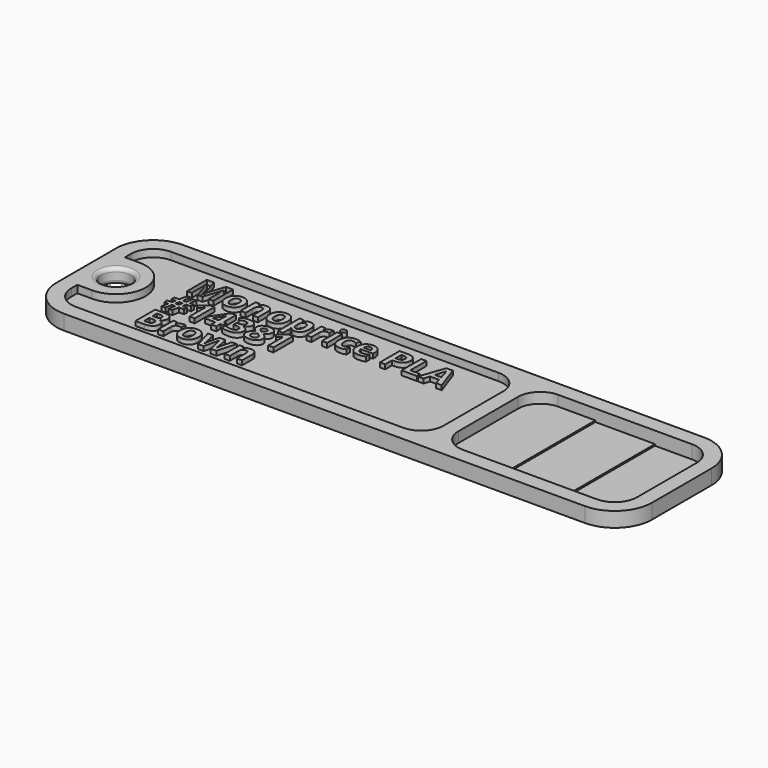
from build123d import *

# Parameters (mm, degrees)
F1_DEPTH      = 2
F3_DEPTH      = 1
F4_R          = 2
F5_DEPTH      = 2.001
F6_R          = 0.5
F7_DEPTH      = 0.4
F9_DEPTH      = 0.2
F11_DEPTH     = 0.2
F12_TEXT_SIZE = 4.6296296296
F13_DEPTH     = 0.6


# Not quite as in the source:
# - Text() gives the source's letters only with a copy of the font that has no kerning and outlines rounded to 1/6400 em; it was checked with that copy


with BuildPart() as f1:
    # F0 (on Top) → F1 (new body)
    with BuildSketch(Plane.XY):
        with BuildLine():
            ThreePointArc((40, 5), (38.5355339059, 8.5355339059), (35, 10))
            Line((35, 10), (-35, 10))
            ThreePointArc((-35, 10), (-38.5355339059, 8.5355339059), (-40, 5))
            Line((-40, 5), (-40, -5))
            ThreePointArc((-40, -5), (-38.5355339059, -8.5355339059), (-35, -10))
            Line((-35, -10), (35, -10))
            ThreePointArc((35, -10), (38.5355339059, -8.5355339059), (40, -5))
            Line((40, -5), (40, 5))
        make_face()
    extrude(amount=F1_DEPTH)

    # F2 (on face) → F3 (cut)
    with BuildSketch(Plane.XY.offset(2)):
        with BuildLine():
            ThreePointArc((35, -8), (37.1213203436, -7.1213203436), (38, -5))
            Line((38, -5), (38, 5))
            ThreePointArc((38, 5), (37.1213203436, 7.1213203436), (35, 8))
            Line((35, 8), (17, 8))
            ThreePointArc((17, 8), (14.8786796564, 7.1213203436), (14, 5))
            Line((14, 5), (14, -5))
            ThreePointArc((14, -5), (14.8786796564, -7.1213203436), (17, -8))
            Line((17, -8), (35, -8))
        make_face()
        with BuildLine():
            ThreePointArc((-38, -5), (-37.1213203436, -7.1213203436), (-35, -8))
            Line((-35, -8), (9, -8))
            ThreePointArc((9, -8), (11.1213203436, -7.1213203436), (12, -5))
            Line((12, -5), (12, 5))
            ThreePointArc((12, 5), (11.1213203436, 7.1213203436), (9, 8))
            Line((9, 8), (-35, 8))
            ThreePointArc((-35, 8), (-37.1213203436, 7.1213203436), (-38, 5))
            Line((-38, 5), (-38, 4))
            Line((-38, 4), (-36, 4))
            ThreePointArc((-36, 4), (-32, 0), (-36, -4))
            Line((-36, -4), (-38, -4))
            Line((-38, -4), (-38, -5))
        make_face()
    extrude(amount=-F3_DEPTH, mode=Mode.SUBTRACT)

    # F4 (on face) → F5 (cut, through all)
    with BuildSketch(Plane.XY.offset(2)):
        with Locations((-36, 0)):
            Circle(F4_R)
    extrude(amount=-F5_DEPTH, mode=Mode.SUBTRACT)

    # F6
    f6_edges = [f1.edges().sort_by_distance(p)[0] for p in [
        (-38, 0, 2),
        (-38, 0, 0),
    ]]
    fillet(f6_edges, radius=F6_R)

    # F7 (cut): a face of the model
    f7_faces = [f1.faces().sort_by_distance(p)[0] for p in [
        (26, 0, 1),
    ]]
    extrude(f7_faces, amount=-F7_DEPTH, mode=Mode.SUBTRACT)

    # F8 (on face) → F9 (cut)
    with BuildSketch(Plane.XY.offset(0.6)):
        with BuildLine():
            Line((22, -8), (35, -8))
            ThreePointArc((35, -8), (37.1213203436, -7.1213203436), (38, -5))
            Line((38, -5), (38, 5))
            ThreePointArc((38, 5), (37.1213203436, 7.1213203436), (35, 8))
            Line((35, 8), (22, 8))
            Line((22, 8), (22, -8))
        make_face()
    extrude(amount=-F9_DEPTH, mode=Mode.SUBTRACT)

    # F10 (on face) → F11 (cut)
    with BuildSketch(Plane.XY.offset(0.4)):
        with BuildLine():
            ThreePointArc((38, 5), (37.1213203436, 7.1213203436), (35, 8))
            Line((35, 8), (30, 8))
            Line((30, 8), (30, -8))
            Line((30, -8), (35, -8))
            ThreePointArc((35, -8), (37.1213203436, -7.1213203436), (38, -5))
            Line((38, -5), (38, 5))
        make_face()
    extrude(amount=-F11_DEPTH, mode=Mode.SUBTRACT)

    # F12 (on face) → F13 (join)
    with BuildSketch(Plane.XY.offset(1)):
        with Locations((-29, 2.6666666667)):
            Text('Monoprice PLA', F12_TEXT_SIZE, font='Open Sans', font_style=FontStyle.BOLD, text_align=(TextAlign.LEFT, TextAlign.BOTTOM))
        with Locations((-29, -1.6666666667)):
            Text('#14381', F12_TEXT_SIZE, font='Open Sans', font_style=FontStyle.BOLD, text_align=(TextAlign.LEFT, TextAlign.BOTTOM))
        with Locations((-29, -6)):
            Text('Brown', F12_TEXT_SIZE, font='Open Sans', font_style=FontStyle.BOLD, text_align=(TextAlign.LEFT, TextAlign.BOTTOM))
    extrude(amount=F13_DEPTH)


solid = f1.part
